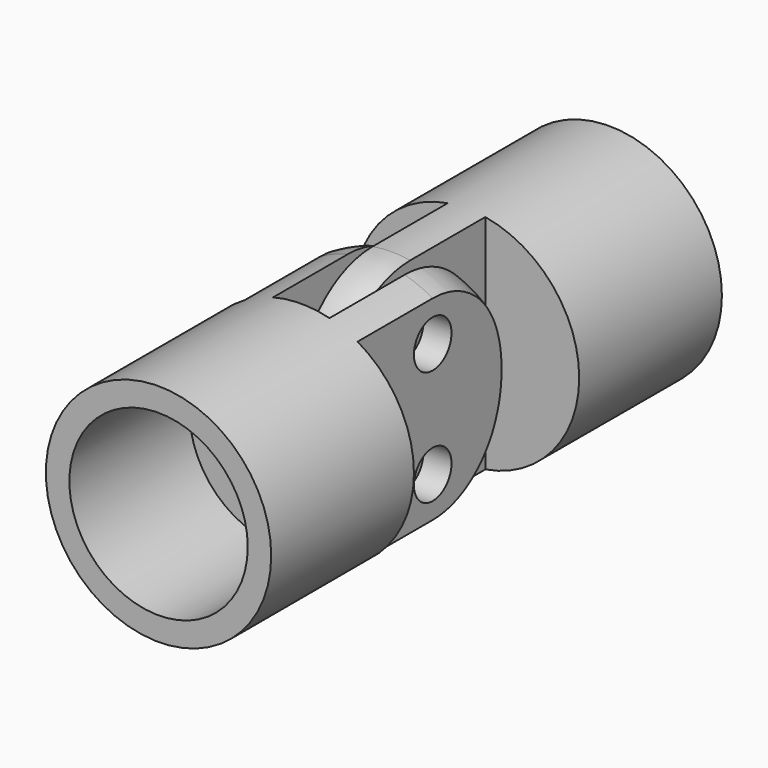
from build123d import *

# Parameters (mm, degrees)
F1_DEPTH       = 12
F2_W           = 18.0606292561
F2_H           = 16.2687138654
F2_R           = 6
F3_DEPTH       = 35.7
F4_R           = 1.25
F5_DEPTH       = 25
F6_R           = 4.75
F7_DEPTH       = 8
F8_R           = 4.75
F9_DEPTH       = 8
F10_T2_ANGLE   = 257.9249090799
F10_T4_ANGLE   = 257.9249090799
F10_2_T2_ANGLE = 254.2577543973
F10_2_T4_ANGLE = 254.2577543973
F10_2_T6_ANGLE = 254.2577543973
F10_2_T8_ANGLE = 254.2577543973
F12_R          = 1.25
F13_DEPTH      = 15


# Not quite as in the source:
# - a fillet or chamfer that OpenCascade refuses, or shapes differently, is made with other operations: its cross-section is extruded or revolved along the edge and cut away or added
# - two fillets or chamfers of one size are made in one step


with BuildPart() as f1:
    # F0 (on Top) → F1 (new body)
    with BuildSketch(Plane.XY):
        Polygon((6, 9.5), (-6, 9.5), (-6, 0), (-1, 0), (-1, -10), (1, -10), (1, 0), (6, 0), align=None)
    extrude(amount=F1_DEPTH)


with BuildPart() as f1b:
    # F0 (on Top) → F1, piece 2 (new body)
    with BuildSketch(Plane.XY):
        Polygon((-6, -11), (-6, -20.5), (6, -20.5), (6, -11), (3, -11), (3, -1), (1.5, -1), (1.5, -11), (-1.5, -11), (-1.5, -1), (-3, -1), (-3, -11), align=None)
    extrude(amount=F1_DEPTH)


with BuildPart() as f3_tool:
    # F2 (on face) → F3 (new body)
    with BuildSketch(Plane.XZ.offset(20.5)):
        with Locations((0.2045785077, 5.5509812664)):
            Rectangle(F2_W, F2_H)
        with Locations((0, 6)):
            Circle(F2_R, mode=Mode.SUBTRACT)
    extrude(amount=-F3_DEPTH)


with BuildPart() as f1_1:
    add(f1.part)

    # F3: cut by f3_tool
    add(f3_tool.part, mode=Mode.SUBTRACT)


with BuildPart() as f1b_1:
    add(f1b.part)

    # F3: cut by f3_tool
    add(f3_tool.part, mode=Mode.SUBTRACT)


with BuildPart() as f5_tool:
    # F4 (on face) → F5 (new body)
    with BuildSketch(Plane.YZ.offset(3)):
        with Locations((-6, 2.9405249807)):
            Circle(F4_R)
    extrude(amount=-F5_DEPTH)


with BuildPart() as f1_2:
    add(f1_1.part)

    # F5: cut by f5_tool
    add(f5_tool.part, mode=Mode.SUBTRACT)

    # F8 (on face) → F9 (cut)
    with BuildSketch(Plane(origin=(0, 9.5, 0), x_dir=(-1, 0, 0), z_dir=(0, 1, 0))):
        with Locations((0, 6)):
            Circle(F8_R)
    extrude(amount=-F9_DEPTH, mode=Mode.SUBTRACT)

    # F10: fillet of radius 5 on 2 edges, made by hand

    # F10_s1 → F10_t2 (revolve, cut)
    with BuildSketch(Plane(origin=(-2.9336228252, 0, 3.6275803689), x_dir=(0, 1, 0), z_dir=(-0.6288109985, 0, 0.7775581831))):
        with BuildLine():
            ThreePointArc((-5, -9.7728659911), (-8.5355339059, -8.308399897), (-10, -4.7728659911))
            Line((-10, -4.7728659911), (-10, -9.7728659911))
            Line((-10, -9.7728659911), (-5, -9.7728659911))
        make_face()
    revolve(axis=Axis((0, -10, 6), (0, 1, 0)), revolution_arc=F10_T2_ANGLE, mode=Mode.SUBTRACT)

    # F10_s3 → F10_t4 (revolve, cut)
    with BuildSketch(Plane(origin=(-2.9336228252, 0, 3.6275803689), x_dir=(0, 1, 0), z_dir=(0.6288109985, 0, -0.7775581831))):
        with BuildLine():
            ThreePointArc((-5, -2.2271340089), (-8.5355339059, -0.7626679148), (-10, 2.7728659911))
            Line((-10, 2.7728659911), (-10, -2.2271340089))
            Line((-10, -2.2271340089), (-5, -2.2271340089))
        make_face()
    revolve(axis=Axis((0, -10, 6), (0, 1, 0)), revolution_arc=F10_T4_ANGLE, mode=Mode.SUBTRACT)


with BuildPart() as f1b_2:
    add(f1b_1.part)

    # F5: cut by f5_tool
    add(f5_tool.part, mode=Mode.SUBTRACT)

    # F6 (on face) → F7 (cut)
    with BuildSketch(Plane.XZ.offset(20.5)):
        with Locations((0, 6)):
            Circle(F6_R)
    extrude(amount=-F7_DEPTH, mode=Mode.SUBTRACT)

    # F10#2: fillet of radius 5 on 4 edges, made by hand

    # F10_2_s1 → F10_2_t2 (revolve, cut)
    with BuildSketch(Plane(origin=(2.6305512341, 0, 1.5577100829), x_dir=(0, 1, 0), z_dir=(-0.8604543293, 0, -0.5095275725))):
        with BuildLine():
            ThreePointArc((-6, 0.8372740241), (-2.4644660941, -0.62719207), (-1, -4.1627259759))
            Line((-1, -4.1627259759), (-1, 0.8372740241))
            Line((-1, 0.8372740241), (-6, 0.8372740241))
        make_face()
    revolve(axis=Axis((0, -1, 6), (0, -1, 0)), revolution_arc=F10_2_T2_ANGLE, mode=Mode.SUBTRACT)

    # F10_2_s3 → F10_2_t4 (revolve, cut)
    with BuildSketch(Plane(origin=(1.4900240777, 0, 5.6038103325), x_dir=(0, 1, 0), z_dir=(-0.2569661675, 0, -0.9664203996))):
        with BuildLine():
            ThreePointArc((-6, 4.4582029949), (-2.4644660941, 2.9937369009), (-1, -0.5417970051))
            Line((-1, -0.5417970051), (-1, 4.4582029949))
            Line((-1, 4.4582029949), (-6, 4.4582029949))
        make_face()
    revolve(axis=Axis((0, -1, 6), (0, -1, 0)), revolution_arc=F10_2_T4_ANGLE, mode=Mode.SUBTRACT)

    # F10_2_s5 → F10_2_t6 (revolve, cut)
    with BuildSketch(Plane(origin=(2.6305512341, 0, 1.5577100829), x_dir=(0, 1, 0), z_dir=(0.8604543293, 0, 0.5095275725))):
        with BuildLine():
            ThreePointArc((-6, 11.1627259759), (-2.4644660941, 9.6982598818), (-1, 6.1627259759))
            Line((-1, 6.1627259759), (-1, 11.1627259759))
            Line((-1, 11.1627259759), (-6, 11.1627259759))
        make_face()
    revolve(axis=Axis((0, -1, 6), (0, -1, 0)), revolution_arc=F10_2_T6_ANGLE, mode=Mode.SUBTRACT)

    # F10_2_s7 → F10_2_t8 (revolve, cut)
    with BuildSketch(Plane(origin=(1.4900240777, 0, 5.6038103325), x_dir=(0, 1, 0), z_dir=(0.2569661675, 0, 0.9664203996))):
        with BuildLine():
            ThreePointArc((-6, 7.5417970051), (-2.4644660941, 6.077330911), (-1, 2.5417970051))
            Line((-1, 2.5417970051), (-1, 7.5417970051))
            Line((-1, 7.5417970051), (-6, 7.5417970051))
        make_face()
    revolve(axis=Axis((0, -1, 6), (0, -1, 0)), revolution_arc=F10_2_T8_ANGLE, mode=Mode.SUBTRACT)


with BuildPart() as f13_tool:
    # F12 (on face) → F13 (new body)
    with BuildSketch(Plane.YZ.offset(3)):
        with Locations((-6, 9.0594750193)):
            Circle(F12_R)
    extrude(amount=-F13_DEPTH)


with BuildPart() as f1_3:
    add(f1_2.part)

    # F13: cut by f13_tool
    add(f13_tool.part, mode=Mode.SUBTRACT)


with BuildPart() as f1b_3:
    add(f1b_2.part)

    # F13: cut by f13_tool
    add(f13_tool.part, mode=Mode.SUBTRACT)


solid = Compound([f1_3.part, f1b_3.part])
